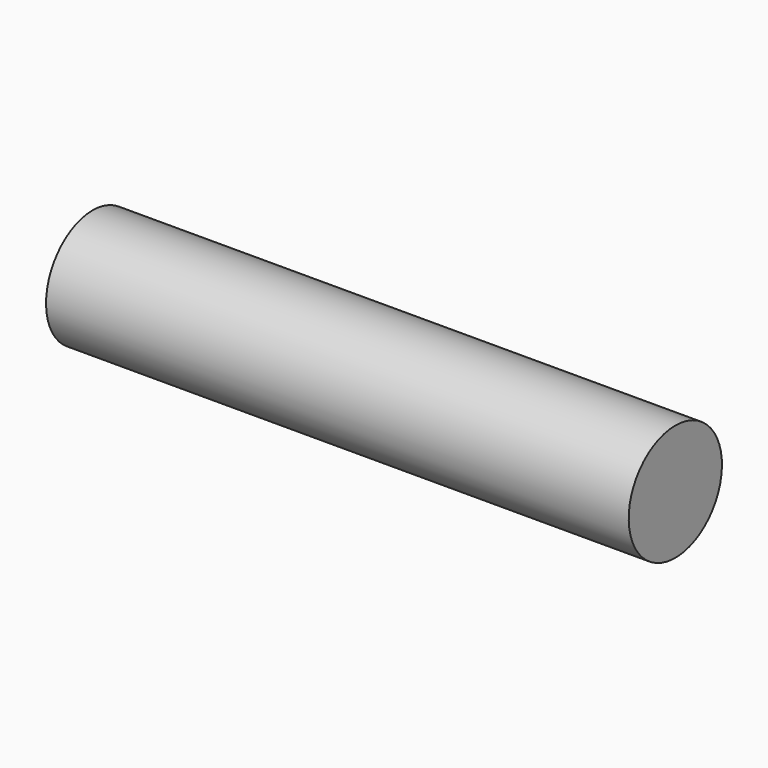
from build123d import *


# Not quite as in the source:
# - ends of sketch curves that miss each other by under 0.0002 mm in the source are joined


with BuildPart() as f1:
    # F0 (on Front) → F1 (revolve)
    with BuildSketch(Plane.XZ):
        Polygon((22.5, 4.4999983363), (0, 4.4999983363), (-22.5, 4.4999983363), (-22.5, -1.6637e-06), (-1.294e-06, -1.6637e-06), (22.5, -1.6637e-06), align=None)
    revolve(axis=Axis((-11.250000647, 0, -1.6637e-06), (1, 0, 0)))


solid = f1.part
